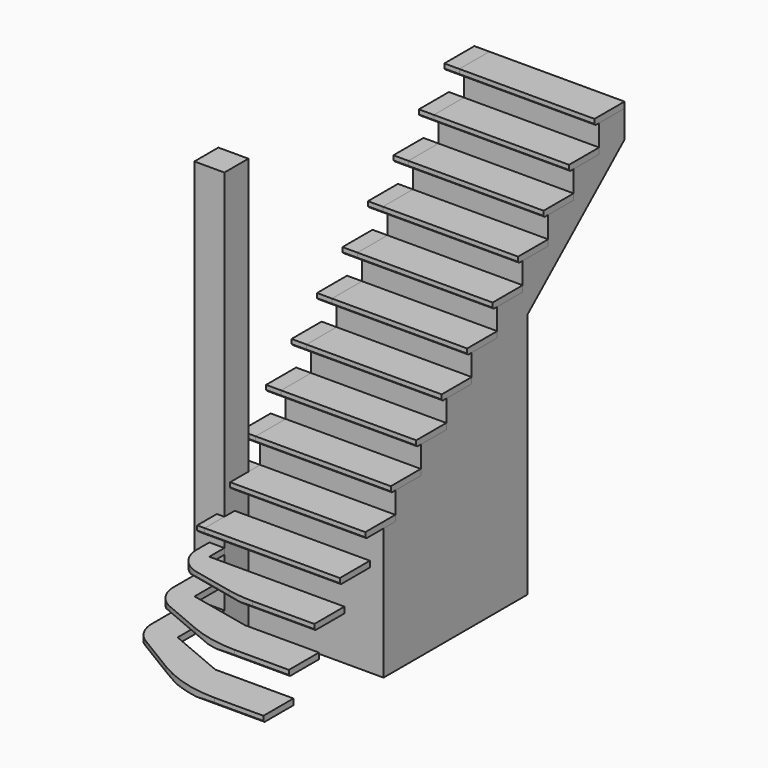
from build123d import *

# Parameters (mm, degrees)
F3_W           = 200
F3_H           = 200
F4_DEPTH       = 2750
F8_DEPTH       = 900
F9_DEPTH       = 100
F11_DEPTH      = 900
F12_DEPTH      = 50
F17_DEPTH      = 40
F19_DEPTH      = 40
F21_DEPTH      = 40
F32_SIZE       = 10
F32_2_SIZE     = 10
F32_3_SIZE     = 10
F32_4_SIZE     = 10
F32_5_SIZE     = 10
F32_6_SIZE     = 10
F32_7_SIZE     = 10
F32_8_SIZE     = 10
F32_9_SIZE     = 10
F32_10_SIZE    = 10
F32_11_SIZE    = 10
F32_12_SIZE    = 10
F32_13_SIZE    = 10
F32_14_SIZE    = 10
F32_15_SIZE    = 10
F32_16_SIZE    = 10
F32_17_SIZE    = 10
F32_18_SIZE    = 10
F32_19_SIZE    = 10
F32_20_SIZE    = 10
F32_21_SIZE    = 10
F32_22_SIZE    = 10
F32_23_SIZE    = 10
F32_24_SIZE    = 10
F34_T1_DEPTH   = 464.801070793
F34_2_T1_DEPTH = 840.9530573364
F34_3_T1_DEPTH = 1149.4231509627
F35_T1_DEPTH   = 833.9140588936
F35_2_T1_DEPTH = 692.872180347
F35_3_T1_DEPTH = 592.6760601916


# Not quite as in the source:
# - a fillet or chamfer that OpenCascade refuses, or shapes differently, is made with other operations: its cross-section is extruded or revolved along the edge and cut away or added
# - a feature of the source that left no trace in its solid (it failed there, or was rolled back) is left out
# - the program builds the solid bodies; features that only make, move or delete a surface that nothing else refers to are left out


with BuildPart() as f4:
    # F3 (on Top) → F4 (new body, through all)
    with BuildSketch(Plane.XY):
        with Locations((-1000, 100)):
            Rectangle(F3_W, F3_H)
    extrude(amount=F4_DEPTH)


with BuildPart() as f8:
    # F7 (on plane+point) → F8 (new body, through all)
    with BuildSketch(Plane.YZ.offset(-900)):
        Polygon((2168, 2562), (1956, 2562), (1956, 2522), (2206, 2522), (2206, 2562), align=None)
    extrude(amount=F8_DEPTH)


with BuildPart() as f8b:
    # F7 (on plane+point) → F8, piece 2 (new body, through all)
    with BuildSketch(Plane.YZ.offset(-900)):
        Polygon((1956, 2379), (1744, 2379), (1744, 2339), (1994, 2339), (1994, 2379), align=None)
    extrude(amount=F8_DEPTH)


with BuildPart() as f8c:
    # F7 (on plane+point) → F8, piece 3 (new body, through all)
    with BuildSketch(Plane.YZ.offset(-900)):
        Polygon((1744, 2196), (1532, 2196), (1532, 2156), (1782, 2156), (1782, 2196), align=None)
    extrude(amount=F8_DEPTH)


with BuildPart() as f8d:
    # F7 (on plane+point) → F8, piece 4 (new body, through all)
    with BuildSketch(Plane.YZ.offset(-900)):
        Polygon((1532, 2013), (1320, 2013), (1320, 1973), (1570, 1973), (1570, 2013), align=None)
    extrude(amount=F8_DEPTH)


with BuildPart() as f8e:
    # F7 (on plane+point) → F8, piece 5 (new body, through all)
    with BuildSketch(Plane.YZ.offset(-900)):
        Polygon((1320, 1830), (1108, 1830), (1108, 1790), (1358, 1790), (1358, 1830), align=None)
    extrude(amount=F8_DEPTH)


with BuildPart() as f8f:
    # F7 (on plane+point) → F8, piece 6 (new body, through all)
    with BuildSketch(Plane.YZ.offset(-900)):
        Polygon((1108, 1647), (896, 1647), (896, 1607), (1146, 1607), (1146, 1647), align=None)
    extrude(amount=F8_DEPTH)


with BuildPart() as f8g:
    # F7 (on plane+point) → F8, piece 7 (new body, through all)
    with BuildSketch(Plane.YZ.offset(-900)):
        Polygon((896, 1464), (684, 1464), (684, 1424), (934, 1424), (934, 1464), align=None)
    extrude(amount=F8_DEPTH)


with BuildPart() as f8h:
    # F7 (on plane+point) → F8, piece 8 (new body, through all)
    with BuildSketch(Plane.YZ.offset(-900)):
        Polygon((684, 1281), (472, 1281), (472, 1241), (722, 1241), (722, 1281), align=None)
    extrude(amount=F8_DEPTH)


with BuildPart() as f8i:
    # F7 (on plane+point) → F8, piece 9 (new body, through all)
    with BuildSketch(Plane.YZ.offset(-900)):
        Polygon((472, 1098), (260, 1098), (260, 1058), (510, 1058), (510, 1098), align=None)
    extrude(amount=F8_DEPTH)


with BuildPart() as f8j:
    # F7 (on plane+point) → F8, piece 10 (new body, through all)
    with BuildSketch(Plane.YZ.offset(-900)):
        Polygon((260, 915), (48, 915), (48, 875), (298, 875), (298, 915), align=None)
    extrude(amount=F8_DEPTH)


with BuildPart() as f8k:
    # F7 (on plane+point) → F8, piece 11 (new body, through all)
    with BuildSketch(Plane.YZ.offset(-900)):
        Polygon((48, 732), (-164, 732), (-164, 692), (86, 692), (86, 732), align=None)
    extrude(amount=F8_DEPTH)


with BuildPart() as f9:
    # F9 (new): a face of the model
    f9_faces = [f8.part.faces().sort_by_distance(p)[0] for p in [
        (-900, 2081, 2542),
    ]]
    extrude(f9_faces, amount=F9_DEPTH)

    # F32#12
    f32_12_edges = [f9.edges().sort_by_distance(p)[0] for p in [
        (-950, 1956, 2522),
    ]]
    chamfer(f32_12_edges, length=F32_12_SIZE)


with BuildPart() as f9b:
    # F9#2 (new): a face of the model
    f9_2_faces = [f8b.part.faces().sort_by_distance(p)[0] for p in [
        (-900, 1869, 2359),
    ]]
    extrude(f9_2_faces, amount=F9_DEPTH)

    # F32#13
    f32_13_edges = [f9b.edges().sort_by_distance(p)[0] for p in [
        (-950, 1744, 2339),
    ]]
    chamfer(f32_13_edges, length=F32_13_SIZE)


with BuildPart() as f9c:
    # F9#3 (new): a face of the model
    f9_3_faces = [f8c.part.faces().sort_by_distance(p)[0] for p in [
        (-900, 1657, 2176),
    ]]
    extrude(f9_3_faces, amount=F9_DEPTH)

    # F32#14
    f32_14_edges = [f9c.edges().sort_by_distance(p)[0] for p in [
        (-950, 1532, 2156),
    ]]
    chamfer(f32_14_edges, length=F32_14_SIZE)


with BuildPart() as f9d:
    # F9#4 (new): a face of the model
    f9_4_faces = [f8d.part.faces().sort_by_distance(p)[0] for p in [
        (-900, 1445, 1993),
    ]]
    extrude(f9_4_faces, amount=F9_DEPTH)

    # F32#15
    f32_15_edges = [f9d.edges().sort_by_distance(p)[0] for p in [
        (-950, 1320, 1973),
    ]]
    chamfer(f32_15_edges, length=F32_15_SIZE)


with BuildPart() as f9e:
    # F9#5 (new): a face of the model
    f9_5_faces = [f8e.part.faces().sort_by_distance(p)[0] for p in [
        (-900, 1233, 1810),
    ]]
    extrude(f9_5_faces, amount=F9_DEPTH)

    # F32#16
    f32_16_edges = [f9e.edges().sort_by_distance(p)[0] for p in [
        (-950, 1108, 1790),
    ]]
    chamfer(f32_16_edges, length=F32_16_SIZE)


with BuildPart() as f9f:
    # F9#6 (new): a face of the model
    f9_6_faces = [f8f.part.faces().sort_by_distance(p)[0] for p in [
        (-900, 1021, 1627),
    ]]
    extrude(f9_6_faces, amount=F9_DEPTH)

    # F32#17
    f32_17_edges = [f9f.edges().sort_by_distance(p)[0] for p in [
        (-950, 896, 1607),
    ]]
    chamfer(f32_17_edges, length=F32_17_SIZE)


with BuildPart() as f9g:
    # F9#7 (new): a face of the model
    f9_7_faces = [f8g.part.faces().sort_by_distance(p)[0] for p in [
        (-900, 809, 1444),
    ]]
    extrude(f9_7_faces, amount=F9_DEPTH)

    # F32#18
    f32_18_edges = [f9g.edges().sort_by_distance(p)[0] for p in [
        (-950, 684, 1424),
    ]]
    chamfer(f32_18_edges, length=F32_18_SIZE)


with BuildPart() as f9h:
    # F9#8 (new): a face of the model
    f9_8_faces = [f8h.part.faces().sort_by_distance(p)[0] for p in [
        (-900, 597, 1261),
    ]]
    extrude(f9_8_faces, amount=F9_DEPTH)

    # F32#19
    f32_19_edges = [f9h.edges().sort_by_distance(p)[0] for p in [
        (-950, 472, 1241),
    ]]
    chamfer(f32_19_edges, length=F32_19_SIZE)


with BuildPart() as f9i:
    # F9#9 (new): a face of the model
    f9_9_faces = [f8i.part.faces().sort_by_distance(p)[0] for p in [
        (-900, 385, 1078),
    ]]
    extrude(f9_9_faces, amount=F9_DEPTH)

    # F32#20
    f32_20_edges = [f9i.edges().sort_by_distance(p)[0] for p in [
        (-950, 260, 1058),
    ]]
    chamfer(f32_20_edges, length=F32_20_SIZE)


with BuildPart() as f9j:
    # F9#10 (new): a face of the model
    f9_10_faces = [f8j.part.faces().sort_by_distance(p)[0] for p in [
        (-900, 173, 895),
    ]]
    extrude(f9_10_faces, amount=F9_DEPTH)


with BuildPart() as f11:
    # F10 (on plane+point) → F11 (new body, through all)
    with BuildSketch(Plane.YZ.offset(-900)):
        Polygon((298, 1058), (298, 915), (298, 875), (200, 875), (200, 0), (1400, 0), (1400, 1643.2547169811), (1146, 1424), (1146, 1607), (934, 1607), (934, 1464), (934, 1424), (722, 1424), (722, 1281), (722, 1241), (510, 1241), (510, 1098), (510, 1058), align=None)
        Polygon((1146, 1424), (1400, 1643.2547169811), (1400, 1973), (1358, 1973), (1358, 1830), (1358, 1790), (1146, 1790), (1146, 1647), (1146, 1607), align=None)
        Polygon((1400, 1973), (1400, 1643.2547169811), (2206, 2339), (2206, 2522), (1994, 2522), (1994, 2379), (1994, 2339), (1782, 2339), (1782, 2196), (1782, 2156), (1570, 2156), (1570, 2013), (1570, 1973), align=None)
    extrude(amount=F11_DEPTH)


with BuildPart() as f12:
    # F12 (new): a face of the model
    f12_faces = [f8k.part.faces().sort_by_distance(p)[0] for p in [
        (-900, -39, 712),
    ]]
    extrude(f12_faces, amount=F12_DEPTH)

    # F32#21
    f32_21_edges = [f12.edges().sort_by_distance(p)[0] for p in [
        (-925, -164, 692),
        (-950, -39, 692),
    ]]
    chamfer(f32_21_edges, length=F32_21_SIZE)


with BuildPart() as f17:
    # F16 (on plane+point) → F17 (new body)
    with BuildSketch(Plane.XY.offset(549)):
        Polygon((-1000, -266), (-500, -376), (0, -376), (0, -126), (-900, -126), (-900, 0), (-1000, 0), (-1000, -126), align=None)
    extrude(amount=-F17_DEPTH)

    # F32#22
    f32_22_edges = [f17.edges().sort_by_distance(p)[0] for p in [
        (-1000, -133, 509),
        (-750, -321, 509),
        (-250, -376, 509),
    ]]
    chamfer(f32_22_edges, length=F32_22_SIZE)

    # F34: fillet of radius 800 on 1 edges, made by hand

    # F34_s2 → F34_t1 (cut)
    with BuildSketch(Plane.XY.offset(301.5994646035)):
        with BuildLine():
            ThreePointArc((-584.9292119815, -357.3155733641), (-499.4907583887, -371.3151761067), (-413.0397858414, -376))
            Line((-413.0397858414, -376), (-500, -376))
            Line((-500, -376), (-584.9292119815, -357.3155733641))
        make_face()
    extrude(amount=F34_T1_DEPTH, mode=Mode.SUBTRACT)

    # F35: fillet of radius 200 on 1 edges, made by hand

    # F35_s2 → F35_t1 (cut)
    with BuildSketch(Plane.XY.offset(117.0429705532)):
        with BuildLine():
            ThreePointArc((-842.972356535, -300.5460815623), (-955.8757057835, -230.5278595406), (-1000, -105.2171882213))
            Line((-1000, -105.2171882213), (-1000, -266))
            Line((-1000, -266), (-842.972356535, -300.5460815623))
        make_face()
    extrude(amount=F35_T1_DEPTH, mode=Mode.SUBTRACT)


with BuildPart() as f19:
    # F18 (on plane+point) → F19 (new body)
    with BuildSketch(Plane.XY.offset(366)):
        Polygon((-1050, -366), (-525, -588), (0, -588), (0, -338), (-490.9090909091, -338), (-900, -248), (-900, 0), (-1050, 0), (-1050, -226), align=None)
    extrude(amount=-F19_DEPTH)

    # F32#23
    f32_23_edges = [f19.edges().sort_by_distance(p)[0] for p in [
        (-1050, -183, 326),
        (-787.5, -477, 326),
        (-262.5, -588, 326),
    ]]
    chamfer(f32_23_edges, length=F32_23_SIZE)

    # F34#2: fillet of radius 800 on 1 edges, made by hand

    # F34_2_s2 → F34_2_t1 (cut)
    with BuildSketch(Plane.XY.offset(-69.4765286682)):
        with BuildLine():
            ThreePointArc((-674.3840204929, -524.8318999059), (-521.7661123215, -572.0489525293), (-362.8093885327, -588))
            Line((-362.8093885327, -588), (-525, -588))
            Line((-525, -588), (-674.3840204929, -524.8318999059))
        make_face()
    extrude(amount=F34_2_T1_DEPTH, mode=Mode.SUBTRACT)

    # F35#2: fillet of radius 200 on 1 edges, made by hand

    # F35_2_s2 → F35_2_t1 (cut)
    with BuildSketch(Plane.XY.offset(4.5639098265)):
        with BuildLine():
            ThreePointArc((-927.89365799, -417.6335389071), (-1016.7014271055, -343.927302383), (-1050, -233.4255639306))
            Line((-1050, -233.4255639306), (-1050, -366))
            Line((-1050, -366), (-927.89365799, -417.6335389071))
        make_face()
    extrude(amount=F35_2_T1_DEPTH, mode=Mode.SUBTRACT)


with BuildPart() as f21:
    # F20 (on plane+point) → F21 (new body)
    with BuildSketch(Plane.XY.offset(183)):
        Polygon((-1100, -466), (-550, -800), (0, -800), (0, -550), (-520.2702702703, -550), (-900, -389.4285714286), (-900, 0), (-1100, 0), (-1100, -326), align=None)
    extrude(amount=-F21_DEPTH)

    # F32#24
    f32_24_edges = [f21.edges().sort_by_distance(p)[0] for p in [
        (-1100, -233, 143),
        (-825, -633, 143),
        (-275, -800, 143),
    ]]
    chamfer(f32_24_edges, length=F32_24_SIZE)

    # F34#3: fillet of radius 800 on 1 edges, made by hand

    # F34_3_s2 → F34_3_t1 (cut)
    with BuildSketch(Plane.XY.offset(-406.7115754813)):
        with BuildLine():
            ThreePointArc((-741.3627609955, -683.7906142318), (-541.7162842473, -770.4000556157), (-326.1153698075, -800))
            Line((-326.1153698075, -800), (-550, -800))
            Line((-550, -800), (-741.3627609955, -683.7906142318))
        make_face()
    extrude(amount=F34_3_T1_DEPTH, mode=Mode.SUBTRACT)

    # F35#3: fillet of radius 200 on 1 edges, made by hand

    # F35_3_s2 → F35_3_t1 (cut)
    with BuildSketch(Plane.XY.offset(-128.3380300958)):
        with BuildLine():
            ThreePointArc((-1003.811847797, -524.4124415196), (-1074.3019930457, -451.5403466922), (-1100, -353.4647879617))
            Line((-1100, -353.4647879617), (-1100, -466))
            Line((-1100, -466), (-1003.811847797, -524.4124415196))
        make_face()
    extrude(amount=F35_3_T1_DEPTH, mode=Mode.SUBTRACT)


with BuildPart() as f8_1:
    add(f8.part)

    # F32
    f32_edges = [f8_1.edges().sort_by_distance(p)[0] for p in [
        (-450, 1956, 2522),
    ]]
    chamfer(f32_edges, length=F32_SIZE)


with BuildPart() as f8b_1:
    add(f8b.part)

    # F32#2
    f32_2_edges = [f8b_1.edges().sort_by_distance(p)[0] for p in [
        (-450, 1744, 2339),
    ]]
    chamfer(f32_2_edges, length=F32_2_SIZE)


with BuildPart() as f8c_1:
    add(f8c.part)

    # F32#3
    f32_3_edges = [f8c_1.edges().sort_by_distance(p)[0] for p in [
        (-450, 1532, 2156),
    ]]
    chamfer(f32_3_edges, length=F32_3_SIZE)


with BuildPart() as f8d_1:
    add(f8d.part)

    # F32#4
    f32_4_edges = [f8d_1.edges().sort_by_distance(p)[0] for p in [
        (-450, 1320, 1973),
    ]]
    chamfer(f32_4_edges, length=F32_4_SIZE)


with BuildPart() as f8e_1:
    add(f8e.part)

    # F32#5
    f32_5_edges = [f8e_1.edges().sort_by_distance(p)[0] for p in [
        (-450, 1108, 1790),
    ]]
    chamfer(f32_5_edges, length=F32_5_SIZE)


with BuildPart() as f8f_1:
    add(f8f.part)

    # F32#6
    f32_6_edges = [f8f_1.edges().sort_by_distance(p)[0] for p in [
        (-450, 896, 1607),
    ]]
    chamfer(f32_6_edges, length=F32_6_SIZE)


with BuildPart() as f8g_1:
    add(f8g.part)

    # F32#7
    f32_7_edges = [f8g_1.edges().sort_by_distance(p)[0] for p in [
        (-450, 684, 1424),
    ]]
    chamfer(f32_7_edges, length=F32_7_SIZE)


with BuildPart() as f8h_1:
    add(f8h.part)

    # F32#8
    f32_8_edges = [f8h_1.edges().sort_by_distance(p)[0] for p in [
        (-450, 472, 1241),
    ]]
    chamfer(f32_8_edges, length=F32_8_SIZE)


with BuildPart() as f8i_1:
    add(f8i.part)

    # F32#9
    f32_9_edges = [f8i_1.edges().sort_by_distance(p)[0] for p in [
        (-450, 260, 1058),
    ]]
    chamfer(f32_9_edges, length=F32_9_SIZE)


with BuildPart() as f8j_1:
    add(f8j.part)

    # F32#10
    f32_10_edges = [f8j_1.edges().sort_by_distance(p)[0] for p in [
        (-450, 48, 875),
    ]]
    chamfer(f32_10_edges, length=F32_10_SIZE)


with BuildPart() as f8k_1:
    add(f8k.part)

    # F32#11
    f32_11_edges = [f8k_1.edges().sort_by_distance(p)[0] for p in [
        (-450, -164, 692),
    ]]
    chamfer(f32_11_edges, length=F32_11_SIZE)


solid = Compound([f4.part, f9.part, f9b.part, f9c.part, f9d.part, f9e.part, f9f.part, f9g.part, f9h.part, f9i.part, f9j.part, f11.part, f12.part, f17.part, f19.part, f21.part, f8_1.part, f8b_1.part, f8c_1.part, f8d_1.part, f8e_1.part, f8f_1.part, f8g_1.part, f8h_1.part, f8i_1.part, f8j_1.part, f8k_1.part])
